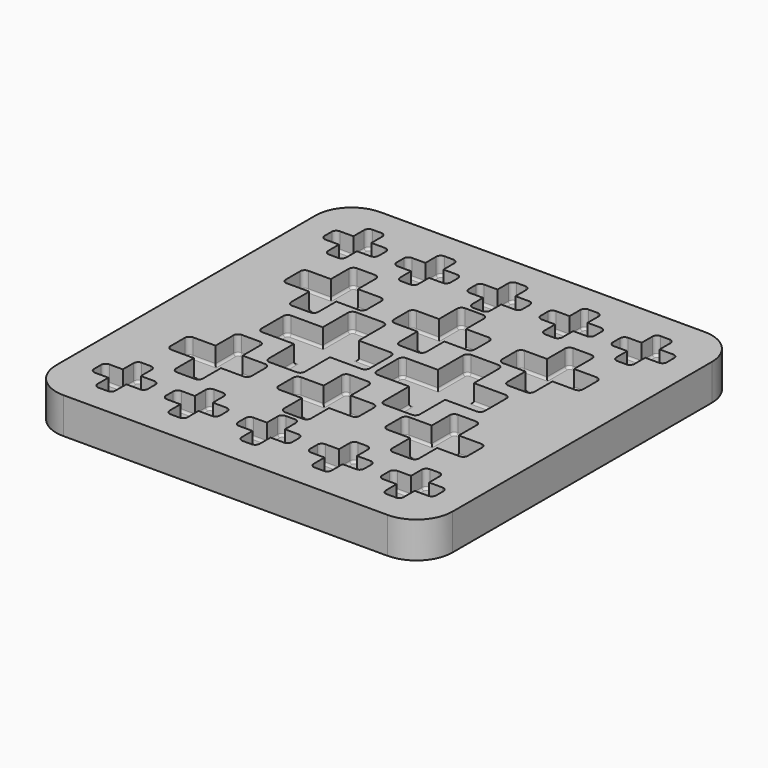
from build123d import *

# Parameters (mm, degrees)
F1_DEPTH = 6.35
F2_W     = 3.175
F2_H     = 3.175
F2_W_2   = 4.7625
F2_H_2   = 4.7625
F2_W_3   = 6.35
F2_H_3   = 6.35
F3_DEPTH = 3.175
F4_R     = 0.396875


with BuildPart() as f1:
    # F0 (on Top) → F1 (new body)
    with BuildSketch(Plane.XY):
        with BuildLine():
            Line((28.575, 34.925), (-28.575, 34.925))
            ThreePointArc((-28.575, 34.925), (-33.0651280605, 33.0651280605), (-34.925, 28.575))
            Line((-34.925, 28.575), (-34.925, -28.575))
            ThreePointArc((-34.925, -28.575), (-33.0651280605, -33.0651280605), (-28.575, -34.925))
            Line((-28.575, -34.925), (28.575, -34.925))
            ThreePointArc((28.575, -34.925), (33.0651280605, -33.0651280605), (34.925, -28.575))
            Line((34.925, -28.575), (34.925, 28.575))
            ThreePointArc((34.925, 28.575), (33.0651280605, 33.0651280605), (28.575, 34.925))
        make_face()
    extrude(amount=F1_DEPTH)

    # F2 (on face) → F3 (cut)
    with BuildSketch(Plane.XY.offset(6.35)):
        with BuildLine():
            ThreePointArc((-23.8125, 29.36875), (-24.0449839924, 29.9300160076), (-24.60625, 30.1625))
            Line((-24.60625, 30.1625), (-26.19375, 30.1625))
            ThreePointArc((-26.19375, 30.1625), (-26.7550160076, 29.9300160076), (-26.9875, 29.36875))
            Line((-26.9875, 29.36875), (-26.9875, 26.9875))
            Line((-26.9875, 26.9875), (-23.8125, 26.9875))
            Line((-23.8125, 26.9875), (-23.8125, 29.36875))
        make_face()
        with BuildLine():
            Line((-21.43125, 26.9875), (-23.8125, 26.9875))
            Line((-23.8125, 26.9875), (-23.8125, 23.8125))
            Line((-23.8125, 23.8125), (-21.43125, 23.8125))
            ThreePointArc((-21.43125, 23.8125), (-20.8699839924, 24.0449839924), (-20.6375, 24.60625))
            Line((-20.6375, 24.60625), (-20.6375, 26.19375))
            ThreePointArc((-20.6375, 26.19375), (-20.8699839924, 26.7550160076), (-21.43125, 26.9875))
        make_face()
        with Locations((-25.4, 25.4)):
            Rectangle(F2_W, F2_H)
        with BuildLine():
            Line((-26.9875, 23.8125), (-26.9875, 26.9875))
            Line((-26.9875, 26.9875), (-29.36875, 26.9875))
            ThreePointArc((-29.36875, 26.9875), (-29.9300160076, 26.7550160076), (-30.1625, 26.19375))
            Line((-30.1625, 26.19375), (-30.1625, 24.60625))
            ThreePointArc((-30.1625, 24.60625), (-29.9300160076, 24.0449839924), (-29.36875, 23.8125))
            Line((-29.36875, 23.8125), (-26.9875, 23.8125))
        make_face()
        with BuildLine():
            Line((-23.8125, 21.43125), (-23.8125, 23.8125))
            Line((-23.8125, 23.8125), (-26.9875, 23.8125))
            Line((-26.9875, 23.8125), (-26.9875, 21.43125))
            ThreePointArc((-26.9875, 21.43125), (-26.7550160076, 20.8699839924), (-26.19375, 20.6375))
            Line((-26.19375, 20.6375), (-24.60625, 20.6375))
            ThreePointArc((-24.60625, 20.6375), (-24.0449839924, 20.8699839924), (-23.8125, 21.43125))
        make_face()
        with BuildLine():
            ThreePointArc((-16.66875, 19.05), (-16.9012339924, 19.6112660076), (-17.4625, 19.84375))
            Line((-17.4625, 19.84375), (-20.6375, 19.84375))
            ThreePointArc((-20.6375, 19.84375), (-21.1987660076, 19.6112660076), (-21.43125, 19.05))
            Line((-21.43125, 19.05), (-21.43125, 15.08125))
            Line((-21.43125, 15.08125), (-16.66875, 15.08125))
            Line((-16.66875, 15.08125), (-16.66875, 19.05))
        make_face()
        with BuildLine():
            Line((-12.7, 15.08125), (-16.66875, 15.08125))
            Line((-16.66875, 15.08125), (-16.66875, 10.31875))
            Line((-16.66875, 10.31875), (-12.7, 10.31875))
            ThreePointArc((-12.7, 10.31875), (-12.1387339924, 10.5512339924), (-11.90625, 11.1125))
            Line((-11.90625, 11.1125), (-11.90625, 14.2875))
            ThreePointArc((-11.90625, 14.2875), (-12.1387339924, 14.8487660076), (-12.7, 15.08125))
        make_face()
        with Locations((-19.05, 12.7)):
            Rectangle(F2_W_2, F2_H_2)
        with BuildLine():
            Line((-21.43125, 10.31875), (-21.43125, 15.08125))
            Line((-21.43125, 15.08125), (-25.4, 15.08125))
            ThreePointArc((-25.4, 15.08125), (-25.9612660076, 14.8487660076), (-26.19375, 14.2875))
            Line((-26.19375, 14.2875), (-26.19375, 11.1125))
            ThreePointArc((-26.19375, 11.1125), (-25.9612660076, 10.5512339924), (-25.4, 10.31875))
            Line((-25.4, 10.31875), (-21.43125, 10.31875))
        make_face()
        with BuildLine():
            Line((-16.66875, 6.35), (-16.66875, 10.31875))
            Line((-16.66875, 10.31875), (-21.43125, 10.31875))
            Line((-21.43125, 10.31875), (-21.43125, 6.35))
            ThreePointArc((-21.43125, 6.35), (-21.1987660076, 5.7887339924), (-20.6375, 5.55625))
            Line((-20.6375, 5.55625), (-17.4625, 5.55625))
            ThreePointArc((-17.4625, 5.55625), (-16.9012339924, 5.7887339924), (-16.66875, 6.35))
        make_face()
        with BuildLine():
            Line((-7.77875, 9.525), (-12.54125, 9.525))
            ThreePointArc((-12.54125, 9.525), (-13.1025160076, 9.2925160076), (-13.335, 8.73125))
            Line((-13.335, 8.73125), (-13.335, 3.175))
            Line((-13.335, 3.175), (-6.985, 3.175))
            Line((-6.985, 3.175), (-6.985, 8.73125))
            ThreePointArc((-6.985, 8.73125), (-7.2174839924, 9.2925160076), (-7.77875, 9.525))
        make_face()
        with Locations((-10.16, 0)):
            Rectangle(F2_W_3, F2_H_3)
        with BuildLine():
            Line((-13.335, -3.175), (-13.335, 3.175))
            Line((-13.335, 3.175), (-18.89125, 3.175))
            ThreePointArc((-18.89125, 3.175), (-19.4525160076, 2.9425160076), (-19.685, 2.38125))
            Line((-19.685, 2.38125), (-19.685, -2.38125))
            ThreePointArc((-19.685, -2.38125), (-19.4525160076, -2.9425160076), (-18.89125, -3.175))
            Line((-18.89125, -3.175), (-13.335, -3.175))
        make_face()
        with BuildLine():
            Line((-1.42875, 3.175), (-6.985, 3.175))
            Line((-6.985, 3.175), (-6.985, -3.175))
            Line((-6.985, -3.175), (-1.42875, -3.175))
            ThreePointArc((-1.42875, -3.175), (-0.8674839924, -2.9425160076), (-0.635, -2.38125))
            Line((-0.635, -2.38125), (-0.635, 2.38125))
            ThreePointArc((-0.635, 2.38125), (-0.8674839924, 2.9425160076), (-1.42875, 3.175))
        make_face()
        with BuildLine():
            Line((-6.985, -3.175), (-13.335, -3.175))
            Line((-13.335, -3.175), (-13.335, -8.73125))
            ThreePointArc((-13.335, -8.73125), (-13.1025160076, -9.2925160076), (-12.54125, -9.525))
            Line((-12.54125, -9.525), (-7.77875, -9.525))
            ThreePointArc((-7.77875, -9.525), (-7.2174839924, -9.2925160076), (-6.985, -8.73125))
            Line((-6.985, -8.73125), (-6.985, -3.175))
        make_face()
        with BuildLine():
            ThreePointArc((-13.49375, 30.1625), (-14.0550160076, 29.9300160076), (-14.2875, 29.36875))
            Line((-14.2875, 29.36875), (-14.2875, 26.9875))
            Line((-14.2875, 26.9875), (-11.1125, 26.9875))
            Line((-11.1125, 26.9875), (-11.1125, 29.36875))
            ThreePointArc((-11.1125, 29.36875), (-11.3449839924, 29.9300160076), (-11.90625, 30.1625))
            Line((-11.90625, 30.1625), (-13.49375, 30.1625))
        make_face()
        with Locations((-12.7, 25.4)):
            Rectangle(F2_W, F2_H)
        with BuildLine():
            Line((-14.2875, 23.8125), (-14.2875, 26.9875))
            Line((-14.2875, 26.9875), (-16.66875, 26.9875))
            ThreePointArc((-16.66875, 26.9875), (-17.2300160076, 26.7550160076), (-17.4625, 26.19375))
            Line((-17.4625, 26.19375), (-17.4625, 24.60625))
            ThreePointArc((-17.4625, 24.60625), (-17.2300160076, 24.0449839924), (-16.66875, 23.8125))
            Line((-16.66875, 23.8125), (-14.2875, 23.8125))
        make_face()
        with BuildLine():
            Line((-11.1125, 23.8125), (-14.2875, 23.8125))
            Line((-14.2875, 23.8125), (-14.2875, 21.43125))
            ThreePointArc((-14.2875, 21.43125), (-14.0550160076, 20.8699839924), (-13.49375, 20.6375))
            Line((-13.49375, 20.6375), (-11.90625, 20.6375))
            ThreePointArc((-11.90625, 20.6375), (-11.3449839924, 20.8699839924), (-11.1125, 21.43125))
            Line((-11.1125, 21.43125), (-11.1125, 23.8125))
        make_face()
        with BuildLine():
            Line((-8.73125, 26.9875), (-11.1125, 26.9875))
            Line((-11.1125, 26.9875), (-11.1125, 23.8125))
            Line((-11.1125, 23.8125), (-8.73125, 23.8125))
            ThreePointArc((-8.73125, 23.8125), (-8.1699839924, 24.0449839924), (-7.9375, 24.60625))
            Line((-7.9375, 24.60625), (-7.9375, 26.19375))
            ThreePointArc((-7.9375, 26.19375), (-8.1699839924, 26.7550160076), (-8.73125, 26.9875))
        make_face()
        with BuildLine():
            ThreePointArc((-0.79375, 30.1625), (-1.3550160076, 29.9300160076), (-1.5875, 29.36875))
            Line((-1.5875, 29.36875), (-1.5875, 26.9875))
            Line((-1.5875, 26.9875), (1.5875, 26.9875))
            Line((1.5875, 26.9875), (1.5875, 29.36875))
            ThreePointArc((1.5875, 29.36875), (1.3550160076, 29.9300160076), (0.79375, 30.1625))
            Line((0.79375, 30.1625), (-0.79375, 30.1625))
        make_face()
        with Locations((0, 25.4)):
            Rectangle(F2_W, F2_H)
        with BuildLine():
            Line((-1.5875, 23.8125), (-1.5875, 26.9875))
            Line((-1.5875, 26.9875), (-3.96875, 26.9875))
            ThreePointArc((-3.96875, 26.9875), (-4.5300160076, 26.7550160076), (-4.7625, 26.19375))
            Line((-4.7625, 26.19375), (-4.7625, 24.60625))
            ThreePointArc((-4.7625, 24.60625), (-4.5300160076, 24.0449839924), (-3.96875, 23.8125))
            Line((-3.96875, 23.8125), (-1.5875, 23.8125))
        make_face()
        with BuildLine():
            Line((1.5875, 23.8125), (-1.5875, 23.8125))
            Line((-1.5875, 23.8125), (-1.5875, 21.43125))
            ThreePointArc((-1.5875, 21.43125), (-1.3550160076, 20.8699839924), (-0.79375, 20.6375))
            Line((-0.79375, 20.6375), (0.79375, 20.6375))
            ThreePointArc((0.79375, 20.6375), (1.3550160076, 20.8699839924), (1.5875, 21.43125))
            Line((1.5875, 21.43125), (1.5875, 23.8125))
        make_face()
        with BuildLine():
            Line((3.96875, 26.9875), (1.5875, 26.9875))
            Line((1.5875, 26.9875), (1.5875, 23.8125))
            Line((1.5875, 23.8125), (3.96875, 23.8125))
            ThreePointArc((3.96875, 23.8125), (4.5300160076, 24.0449839924), (4.7625, 24.60625))
            Line((4.7625, 24.60625), (4.7625, 26.19375))
            ThreePointArc((4.7625, 26.19375), (4.5300160076, 26.7550160076), (3.96875, 26.9875))
        make_face()
        with BuildLine():
            ThreePointArc((11.90625, 30.1625), (11.3449839924, 29.9300160076), (11.1125, 29.36875))
            Line((11.1125, 29.36875), (11.1125, 26.9875))
            Line((11.1125, 26.9875), (14.2875, 26.9875))
            Line((14.2875, 26.9875), (14.2875, 29.36875))
            ThreePointArc((14.2875, 29.36875), (14.0550160076, 29.9300160076), (13.49375, 30.1625))
            Line((13.49375, 30.1625), (11.90625, 30.1625))
        make_face()
        with Locations((12.7, 25.4)):
            Rectangle(F2_W, F2_H)
        with BuildLine():
            Line((11.1125, 23.8125), (11.1125, 26.9875))
            Line((11.1125, 26.9875), (8.73125, 26.9875))
            ThreePointArc((8.73125, 26.9875), (8.1699839924, 26.7550160076), (7.9375, 26.19375))
            Line((7.9375, 26.19375), (7.9375, 24.60625))
            ThreePointArc((7.9375, 24.60625), (8.1699839924, 24.0449839924), (8.73125, 23.8125))
            Line((8.73125, 23.8125), (11.1125, 23.8125))
        make_face()
        with BuildLine():
            Line((14.2875, 23.8125), (11.1125, 23.8125))
            Line((11.1125, 23.8125), (11.1125, 21.43125))
            ThreePointArc((11.1125, 21.43125), (11.3449839924, 20.8699839924), (11.90625, 20.6375))
            Line((11.90625, 20.6375), (13.49375, 20.6375))
            ThreePointArc((13.49375, 20.6375), (14.0550160076, 20.8699839924), (14.2875, 21.43125))
            Line((14.2875, 21.43125), (14.2875, 23.8125))
        make_face()
        with BuildLine():
            Line((16.66875, 26.9875), (14.2875, 26.9875))
            Line((14.2875, 26.9875), (14.2875, 23.8125))
            Line((14.2875, 23.8125), (16.66875, 23.8125))
            ThreePointArc((16.66875, 23.8125), (17.2300160076, 24.0449839924), (17.4625, 24.60625))
            Line((17.4625, 24.60625), (17.4625, 26.19375))
            ThreePointArc((17.4625, 26.19375), (17.2300160076, 26.7550160076), (16.66875, 26.9875))
        make_face()
        with BuildLine():
            ThreePointArc((24.60625, 30.1625), (24.0449839924, 29.9300160076), (23.8125, 29.36875))
            Line((23.8125, 29.36875), (23.8125, 26.9875))
            Line((23.8125, 26.9875), (26.9875, 26.9875))
            Line((26.9875, 26.9875), (26.9875, 29.36875))
            ThreePointArc((26.9875, 29.36875), (26.7550160076, 29.9300160076), (26.19375, 30.1625))
            Line((26.19375, 30.1625), (24.60625, 30.1625))
        make_face()
        with Locations((25.4, 25.4)):
            Rectangle(F2_W, F2_H)
        with BuildLine():
            Line((23.8125, 23.8125), (23.8125, 26.9875))
            Line((23.8125, 26.9875), (21.43125, 26.9875))
            ThreePointArc((21.43125, 26.9875), (20.8699839924, 26.7550160076), (20.6375, 26.19375))
            Line((20.6375, 26.19375), (20.6375, 24.60625))
            ThreePointArc((20.6375, 24.60625), (20.8699839924, 24.0449839924), (21.43125, 23.8125))
            Line((21.43125, 23.8125), (23.8125, 23.8125))
        make_face()
        with BuildLine():
            Line((26.9875, 23.8125), (23.8125, 23.8125))
            Line((23.8125, 23.8125), (23.8125, 21.43125))
            ThreePointArc((23.8125, 21.43125), (24.0449839924, 20.8699839924), (24.60625, 20.6375))
            Line((24.60625, 20.6375), (26.19375, 20.6375))
            ThreePointArc((26.19375, 20.6375), (26.7550160076, 20.8699839924), (26.9875, 21.43125))
            Line((26.9875, 21.43125), (26.9875, 23.8125))
        make_face()
        with BuildLine():
            Line((29.36875, 26.9875), (26.9875, 26.9875))
            Line((26.9875, 26.9875), (26.9875, 23.8125))
            Line((26.9875, 23.8125), (29.36875, 23.8125))
            ThreePointArc((29.36875, 23.8125), (29.9300160076, 24.0449839924), (30.1625, 24.60625))
            Line((30.1625, 24.60625), (30.1625, 26.19375))
            ThreePointArc((30.1625, 26.19375), (29.9300160076, 26.7550160076), (29.36875, 26.9875))
        make_face()
        with BuildLine():
            Line((-1.5875, 5.55625), (1.5875, 5.55625))
            ThreePointArc((1.5875, 5.55625), (2.1487660076, 5.7887339924), (2.38125, 6.35))
            Line((2.38125, 6.35), (2.38125, 10.31875))
            Line((2.38125, 10.31875), (-2.38125, 10.31875))
            Line((-2.38125, 10.31875), (-2.38125, 6.35))
            ThreePointArc((-2.38125, 6.35), (-2.1487660076, 5.7887339924), (-1.5875, 5.55625))
        make_face()
        with BuildLine():
            Line((2.38125, 15.08125), (2.38125, 10.31875))
            Line((2.38125, 10.31875), (6.35, 10.31875))
            ThreePointArc((6.35, 10.31875), (6.9112660076, 10.5512339924), (7.14375, 11.1125))
            Line((7.14375, 11.1125), (7.14375, 14.2875))
            ThreePointArc((7.14375, 14.2875), (6.9112660076, 14.8487660076), (6.35, 15.08125))
            Line((6.35, 15.08125), (2.38125, 15.08125))
        make_face()
        with Locations((0, 12.7)):
            Rectangle(F2_W_2, F2_H_2)
        with BuildLine():
            Line((-6.35, 10.31875), (-2.38125, 10.31875))
            Line((-2.38125, 10.31875), (-2.38125, 15.08125))
            Line((-2.38125, 15.08125), (-6.35, 15.08125))
            ThreePointArc((-6.35, 15.08125), (-6.9112660076, 14.8487660076), (-7.14375, 14.2875))
            Line((-7.14375, 14.2875), (-7.14375, 11.1125))
            ThreePointArc((-7.14375, 11.1125), (-6.9112660076, 10.5512339924), (-6.35, 10.31875))
        make_face()
        with BuildLine():
            Line((-2.38125, 15.08125), (2.38125, 15.08125))
            Line((2.38125, 15.08125), (2.38125, 19.05))
            ThreePointArc((2.38125, 19.05), (2.1487660076, 19.6112660076), (1.5875, 19.84375))
            Line((1.5875, 19.84375), (-1.5875, 19.84375))
            ThreePointArc((-1.5875, 19.84375), (-2.1487660076, 19.6112660076), (-2.38125, 19.05))
            Line((-2.38125, 19.05), (-2.38125, 15.08125))
        make_face()
        with BuildLine():
            Line((17.4625, 5.55625), (20.6375, 5.55625))
            ThreePointArc((20.6375, 5.55625), (21.1987660076, 5.7887339924), (21.43125, 6.35))
            Line((21.43125, 6.35), (21.43125, 10.31875))
            Line((21.43125, 10.31875), (16.66875, 10.31875))
            Line((16.66875, 10.31875), (16.66875, 6.35))
            ThreePointArc((16.66875, 6.35), (16.9012339924, 5.7887339924), (17.4625, 5.55625))
        make_face()
        with BuildLine():
            Line((21.43125, 15.08125), (21.43125, 10.31875))
            Line((21.43125, 10.31875), (25.4, 10.31875))
            ThreePointArc((25.4, 10.31875), (25.9612660076, 10.5512339924), (26.19375, 11.1125))
            Line((26.19375, 11.1125), (26.19375, 14.2875))
            ThreePointArc((26.19375, 14.2875), (25.9612660076, 14.8487660076), (25.4, 15.08125))
            Line((25.4, 15.08125), (21.43125, 15.08125))
        make_face()
        with Locations((19.05, 12.7)):
            Rectangle(F2_W_2, F2_H_2)
        with BuildLine():
            Line((12.7, 10.31875), (16.66875, 10.31875))
            Line((16.66875, 10.31875), (16.66875, 15.08125))
            Line((16.66875, 15.08125), (12.7, 15.08125))
            ThreePointArc((12.7, 15.08125), (12.1387339924, 14.8487660076), (11.90625, 14.2875))
            Line((11.90625, 14.2875), (11.90625, 11.1125))
            ThreePointArc((11.90625, 11.1125), (12.1387339924, 10.5512339924), (12.7, 10.31875))
        make_face()
        with BuildLine():
            Line((16.66875, 15.08125), (21.43125, 15.08125))
            Line((21.43125, 15.08125), (21.43125, 19.05))
            ThreePointArc((21.43125, 19.05), (21.1987660076, 19.6112660076), (20.6375, 19.84375))
            Line((20.6375, 19.84375), (17.4625, 19.84375))
            ThreePointArc((17.4625, 19.84375), (16.9012339924, 19.6112660076), (16.66875, 19.05))
            Line((16.66875, 19.05), (16.66875, 15.08125))
        make_face()
        with BuildLine():
            Line((13.3096, 3.175), (13.3096, 8.73125))
            ThreePointArc((13.3096, 8.73125), (13.0771160076, 9.2925160076), (12.51585, 9.525))
            Line((12.51585, 9.525), (7.75335, 9.525))
            ThreePointArc((7.75335, 9.525), (7.1920839924, 9.2925160076), (6.9596, 8.73125))
            Line((6.9596, 8.73125), (6.9596, 3.175))
            Line((6.9596, 3.175), (13.3096, 3.175))
        make_face()
        with BuildLine():
            Line((18.86585, 3.175), (13.3096, 3.175))
            Line((13.3096, 3.175), (13.3096, -3.175))
            Line((13.3096, -3.175), (18.86585, -3.175))
            ThreePointArc((18.86585, -3.175), (19.4271160076, -2.9425160076), (19.6596, -2.38125))
            Line((19.6596, -2.38125), (19.6596, 2.38125))
            ThreePointArc((19.6596, 2.38125), (19.4271160076, 2.9425160076), (18.86585, 3.175))
        make_face()
        with Locations((10.1346, 0)):
            Rectangle(F2_W_3, F2_H_3)
        with BuildLine():
            Line((13.3096, -8.73125), (13.3096, -3.175))
            Line((13.3096, -3.175), (6.9596, -3.175))
            Line((6.9596, -3.175), (6.9596, -8.73125))
            ThreePointArc((6.9596, -8.73125), (7.1920839924, -9.2925160076), (7.75335, -9.525))
            Line((7.75335, -9.525), (12.51585, -9.525))
            ThreePointArc((12.51585, -9.525), (13.0771160076, -9.2925160076), (13.3096, -8.73125))
        make_face()
        with BuildLine():
            Line((6.9596, -3.175), (6.9596, 3.175))
            Line((6.9596, 3.175), (1.40335, 3.175))
            ThreePointArc((1.40335, 3.175), (0.8420839924, 2.9425160076), (0.6096, 2.38125))
            Line((0.6096, 2.38125), (0.6096, -2.38125))
            ThreePointArc((0.6096, -2.38125), (0.8420839924, -2.9425160076), (1.40335, -3.175))
            Line((1.40335, -3.175), (6.9596, -3.175))
        make_face()
        with BuildLine():
            ThreePointArc((-25.4, -10.31875), (-25.9612660076, -10.5512339924), (-26.19375, -11.1125))
            Line((-26.19375, -11.1125), (-26.19375, -14.2875))
            ThreePointArc((-26.19375, -14.2875), (-25.9612660076, -14.8487660076), (-25.4, -15.08125))
            Line((-25.4, -15.08125), (-21.43125, -15.08125))
            Line((-21.43125, -15.08125), (-21.43125, -10.31875))
            Line((-21.43125, -10.31875), (-25.4, -10.31875))
        make_face()
        with BuildLine():
            Line((-21.43125, -6.35), (-21.43125, -10.31875))
            Line((-21.43125, -10.31875), (-16.66875, -10.31875))
            Line((-16.66875, -10.31875), (-16.66875, -6.35))
            ThreePointArc((-16.66875, -6.35), (-16.9012339924, -5.7887339924), (-17.4625, -5.55625))
            Line((-17.4625, -5.55625), (-20.6375, -5.55625))
            ThreePointArc((-20.6375, -5.55625), (-21.1987660076, -5.7887339924), (-21.43125, -6.35))
        make_face()
        with Locations((-19.05, -12.7)):
            Rectangle(F2_W_2, F2_H_2)
        with BuildLine():
            Line((-12.7, -10.31875), (-16.66875, -10.31875))
            Line((-16.66875, -10.31875), (-16.66875, -15.08125))
            Line((-16.66875, -15.08125), (-12.7, -15.08125))
            ThreePointArc((-12.7, -15.08125), (-12.1387339924, -14.8487660076), (-11.90625, -14.2875))
            Line((-11.90625, -14.2875), (-11.90625, -11.1125))
            ThreePointArc((-11.90625, -11.1125), (-12.1387339924, -10.5512339924), (-12.7, -10.31875))
        make_face()
        with BuildLine():
            Line((-16.66875, -15.08125), (-21.43125, -15.08125))
            Line((-21.43125, -15.08125), (-21.43125, -19.05))
            ThreePointArc((-21.43125, -19.05), (-21.1987660076, -19.6112660076), (-20.6375, -19.84375))
            Line((-20.6375, -19.84375), (-17.4625, -19.84375))
            ThreePointArc((-17.4625, -19.84375), (-16.9012339924, -19.6112660076), (-16.66875, -19.05))
            Line((-16.66875, -19.05), (-16.66875, -15.08125))
        make_face()
        with BuildLine():
            ThreePointArc((-26.9875, -29.36875), (-26.7550160076, -29.9300160076), (-26.19375, -30.1625))
            Line((-26.19375, -30.1625), (-24.60625, -30.1625))
            ThreePointArc((-24.60625, -30.1625), (-24.0449839924, -29.9300160076), (-23.8125, -29.36875))
            Line((-23.8125, -29.36875), (-23.8125, -26.9875))
            Line((-23.8125, -26.9875), (-26.9875, -26.9875))
            Line((-26.9875, -26.9875), (-26.9875, -29.36875))
        make_face()
        with Locations((-25.4, -25.4)):
            Rectangle(F2_W, F2_H)
        with BuildLine():
            Line((-29.36875, -26.9875), (-26.9875, -26.9875))
            Line((-26.9875, -26.9875), (-26.9875, -23.8125))
            Line((-26.9875, -23.8125), (-29.36875, -23.8125))
            ThreePointArc((-29.36875, -23.8125), (-29.9300160076, -24.0449839924), (-30.1625, -24.60625))
            Line((-30.1625, -24.60625), (-30.1625, -26.19375))
            ThreePointArc((-30.1625, -26.19375), (-29.9300160076, -26.7550160076), (-29.36875, -26.9875))
        make_face()
        with BuildLine():
            Line((-23.8125, -23.8125), (-23.8125, -26.9875))
            Line((-23.8125, -26.9875), (-21.43125, -26.9875))
            ThreePointArc((-21.43125, -26.9875), (-20.8699839924, -26.7550160076), (-20.6375, -26.19375))
            Line((-20.6375, -26.19375), (-20.6375, -24.60625))
            ThreePointArc((-20.6375, -24.60625), (-20.8699839924, -24.0449839924), (-21.43125, -23.8125))
            Line((-21.43125, -23.8125), (-23.8125, -23.8125))
        make_face()
        with BuildLine():
            Line((-26.9875, -21.43125), (-26.9875, -23.8125))
            Line((-26.9875, -23.8125), (-23.8125, -23.8125))
            Line((-23.8125, -23.8125), (-23.8125, -21.43125))
            ThreePointArc((-23.8125, -21.43125), (-24.0449839924, -20.8699839924), (-24.60625, -20.6375))
            Line((-24.60625, -20.6375), (-26.19375, -20.6375))
            ThreePointArc((-26.19375, -20.6375), (-26.7550160076, -20.8699839924), (-26.9875, -21.43125))
        make_face()
        with BuildLine():
            ThreePointArc((-11.90625, -30.1625), (-11.3449839924, -29.9300160076), (-11.1125, -29.36875))
            Line((-11.1125, -29.36875), (-11.1125, -26.9875))
            Line((-11.1125, -26.9875), (-14.2875, -26.9875))
            Line((-14.2875, -26.9875), (-14.2875, -29.36875))
            ThreePointArc((-14.2875, -29.36875), (-14.0550160076, -29.9300160076), (-13.49375, -30.1625))
            Line((-13.49375, -30.1625), (-11.90625, -30.1625))
        make_face()
        with Locations((-12.7, -25.4)):
            Rectangle(F2_W, F2_H)
        with BuildLine():
            Line((-11.1125, -23.8125), (-11.1125, -26.9875))
            Line((-11.1125, -26.9875), (-8.73125, -26.9875))
            ThreePointArc((-8.73125, -26.9875), (-8.1699839924, -26.7550160076), (-7.9375, -26.19375))
            Line((-7.9375, -26.19375), (-7.9375, -24.60625))
            ThreePointArc((-7.9375, -24.60625), (-8.1699839924, -24.0449839924), (-8.73125, -23.8125))
            Line((-8.73125, -23.8125), (-11.1125, -23.8125))
        make_face()
        with BuildLine():
            Line((-14.2875, -23.8125), (-11.1125, -23.8125))
            Line((-11.1125, -23.8125), (-11.1125, -21.43125))
            ThreePointArc((-11.1125, -21.43125), (-11.3449839924, -20.8699839924), (-11.90625, -20.6375))
            Line((-11.90625, -20.6375), (-13.49375, -20.6375))
            ThreePointArc((-13.49375, -20.6375), (-14.0550160076, -20.8699839924), (-14.2875, -21.43125))
            Line((-14.2875, -21.43125), (-14.2875, -23.8125))
        make_face()
        with BuildLine():
            Line((-16.66875, -26.9875), (-14.2875, -26.9875))
            Line((-14.2875, -26.9875), (-14.2875, -23.8125))
            Line((-14.2875, -23.8125), (-16.66875, -23.8125))
            ThreePointArc((-16.66875, -23.8125), (-17.2300160076, -24.0449839924), (-17.4625, -24.60625))
            Line((-17.4625, -24.60625), (-17.4625, -26.19375))
            ThreePointArc((-17.4625, -26.19375), (-17.2300160076, -26.7550160076), (-16.66875, -26.9875))
        make_face()
        with BuildLine():
            ThreePointArc((30.1625, -24.60625), (29.9300160076, -24.0449839924), (29.36875, -23.8125))
            Line((29.36875, -23.8125), (26.9875, -23.8125))
            Line((26.9875, -23.8125), (26.9875, -26.9875))
            Line((26.9875, -26.9875), (29.36875, -26.9875))
            ThreePointArc((29.36875, -26.9875), (29.9300160076, -26.7550160076), (30.1625, -26.19375))
            Line((30.1625, -26.19375), (30.1625, -24.60625))
        make_face()
        with Locations((25.4, -25.4)):
            Rectangle(F2_W, F2_H)
        with BuildLine():
            Line((23.8125, -23.8125), (26.9875, -23.8125))
            Line((26.9875, -23.8125), (26.9875, -21.43125))
            ThreePointArc((26.9875, -21.43125), (26.7550160076, -20.8699839924), (26.19375, -20.6375))
            Line((26.19375, -20.6375), (24.60625, -20.6375))
            ThreePointArc((24.60625, -20.6375), (24.0449839924, -20.8699839924), (23.8125, -21.43125))
            Line((23.8125, -21.43125), (23.8125, -23.8125))
        make_face()
        with BuildLine():
            Line((23.8125, -26.9875), (23.8125, -23.8125))
            Line((23.8125, -23.8125), (21.43125, -23.8125))
            ThreePointArc((21.43125, -23.8125), (20.8699839924, -24.0449839924), (20.6375, -24.60625))
            Line((20.6375, -24.60625), (20.6375, -26.19375))
            ThreePointArc((20.6375, -26.19375), (20.8699839924, -26.7550160076), (21.43125, -26.9875))
            Line((21.43125, -26.9875), (23.8125, -26.9875))
        make_face()
        with BuildLine():
            Line((26.9875, -29.36875), (26.9875, -26.9875))
            Line((26.9875, -26.9875), (23.8125, -26.9875))
            Line((23.8125, -26.9875), (23.8125, -29.36875))
            ThreePointArc((23.8125, -29.36875), (24.0449839924, -29.9300160076), (24.60625, -30.1625))
            Line((24.60625, -30.1625), (26.19375, -30.1625))
            ThreePointArc((26.19375, -30.1625), (26.7550160076, -29.9300160076), (26.9875, -29.36875))
        make_face()
        with BuildLine():
            ThreePointArc((-2.38125, -19.05), (-2.1487660076, -19.6112660076), (-1.5875, -19.84375))
            Line((-1.5875, -19.84375), (1.5875, -19.84375))
            ThreePointArc((1.5875, -19.84375), (2.1487660076, -19.6112660076), (2.38125, -19.05))
            Line((2.38125, -19.05), (2.38125, -15.08125))
            Line((2.38125, -15.08125), (-2.38125, -15.08125))
            Line((-2.38125, -15.08125), (-2.38125, -19.05))
        make_face()
        with Locations((0, -12.7)):
            Rectangle(F2_W_2, F2_H_2)
        with BuildLine():
            Line((-6.35, -15.08125), (-2.38125, -15.08125))
            Line((-2.38125, -15.08125), (-2.38125, -10.31875))
            Line((-2.38125, -10.31875), (-6.35, -10.31875))
            ThreePointArc((-6.35, -10.31875), (-6.9112660076, -10.5512339924), (-7.14375, -11.1125))
            Line((-7.14375, -11.1125), (-7.14375, -14.2875))
            ThreePointArc((-7.14375, -14.2875), (-6.9112660076, -14.8487660076), (-6.35, -15.08125))
        make_face()
        with BuildLine():
            Line((2.38125, -10.31875), (2.38125, -15.08125))
            Line((2.38125, -15.08125), (6.35, -15.08125))
            ThreePointArc((6.35, -15.08125), (6.9112660076, -14.8487660076), (7.14375, -14.2875))
            Line((7.14375, -14.2875), (7.14375, -11.1125))
            ThreePointArc((7.14375, -11.1125), (6.9112660076, -10.5512339924), (6.35, -10.31875))
            Line((6.35, -10.31875), (2.38125, -10.31875))
        make_face()
        with BuildLine():
            Line((-2.38125, -6.35), (-2.38125, -10.31875))
            Line((-2.38125, -10.31875), (2.38125, -10.31875))
            Line((2.38125, -10.31875), (2.38125, -6.35))
            ThreePointArc((2.38125, -6.35), (2.1487660076, -5.7887339924), (1.5875, -5.55625))
            Line((1.5875, -5.55625), (-1.5875, -5.55625))
            ThreePointArc((-1.5875, -5.55625), (-2.1487660076, -5.7887339924), (-2.38125, -6.35))
        make_face()
        with BuildLine():
            ThreePointArc((11.1125, -29.36875), (11.3449839924, -29.9300160076), (11.90625, -30.1625))
            Line((11.90625, -30.1625), (13.49375, -30.1625))
            ThreePointArc((13.49375, -30.1625), (14.0550160076, -29.9300160076), (14.2875, -29.36875))
            Line((14.2875, -29.36875), (14.2875, -26.9875))
            Line((14.2875, -26.9875), (11.1125, -26.9875))
            Line((11.1125, -26.9875), (11.1125, -29.36875))
        make_face()
        with Locations((12.7, -25.4)):
            Rectangle(F2_W, F2_H)
        with BuildLine():
            Line((8.73125, -26.9875), (11.1125, -26.9875))
            Line((11.1125, -26.9875), (11.1125, -23.8125))
            Line((11.1125, -23.8125), (8.73125, -23.8125))
            ThreePointArc((8.73125, -23.8125), (8.1699839924, -24.0449839924), (7.9375, -24.60625))
            Line((7.9375, -24.60625), (7.9375, -26.19375))
            ThreePointArc((7.9375, -26.19375), (8.1699839924, -26.7550160076), (8.73125, -26.9875))
        make_face()
        with BuildLine():
            Line((14.2875, -23.8125), (14.2875, -26.9875))
            Line((14.2875, -26.9875), (16.66875, -26.9875))
            ThreePointArc((16.66875, -26.9875), (17.2300160076, -26.7550160076), (17.4625, -26.19375))
            Line((17.4625, -26.19375), (17.4625, -24.60625))
            ThreePointArc((17.4625, -24.60625), (17.2300160076, -24.0449839924), (16.66875, -23.8125))
            Line((16.66875, -23.8125), (14.2875, -23.8125))
        make_face()
        with BuildLine():
            Line((11.1125, -21.43125), (11.1125, -23.8125))
            Line((11.1125, -23.8125), (14.2875, -23.8125))
            Line((14.2875, -23.8125), (14.2875, -21.43125))
            ThreePointArc((14.2875, -21.43125), (14.0550160076, -20.8699839924), (13.49375, -20.6375))
            Line((13.49375, -20.6375), (11.90625, -20.6375))
            ThreePointArc((11.90625, -20.6375), (11.3449839924, -20.8699839924), (11.1125, -21.43125))
        make_face()
        with BuildLine():
            ThreePointArc((-1.5875, -29.36875), (-1.3550160076, -29.9300160076), (-0.79375, -30.1625))
            Line((-0.79375, -30.1625), (0.79375, -30.1625))
            ThreePointArc((0.79375, -30.1625), (1.3550160076, -29.9300160076), (1.5875, -29.36875))
            Line((1.5875, -29.36875), (1.5875, -26.9875))
            Line((1.5875, -26.9875), (-1.5875, -26.9875))
            Line((-1.5875, -26.9875), (-1.5875, -29.36875))
        make_face()
        with BuildLine():
            Line((-3.96875, -26.9875), (-1.5875, -26.9875))
            Line((-1.5875, -26.9875), (-1.5875, -23.8125))
            Line((-1.5875, -23.8125), (-3.96875, -23.8125))
            ThreePointArc((-3.96875, -23.8125), (-4.5300160076, -24.0449839924), (-4.7625, -24.60625))
            Line((-4.7625, -24.60625), (-4.7625, -26.19375))
            ThreePointArc((-4.7625, -26.19375), (-4.5300160076, -26.7550160076), (-3.96875, -26.9875))
        make_face()
        with Locations((0, -25.4)):
            Rectangle(F2_W, F2_H)
        with BuildLine():
            Line((-1.5875, -21.43125), (-1.5875, -23.8125))
            Line((-1.5875, -23.8125), (1.5875, -23.8125))
            Line((1.5875, -23.8125), (1.5875, -21.43125))
            ThreePointArc((1.5875, -21.43125), (1.3550160076, -20.8699839924), (0.79375, -20.6375))
            Line((0.79375, -20.6375), (-0.79375, -20.6375))
            ThreePointArc((-0.79375, -20.6375), (-1.3550160076, -20.8699839924), (-1.5875, -21.43125))
        make_face()
        with BuildLine():
            Line((1.5875, -23.8125), (1.5875, -26.9875))
            Line((1.5875, -26.9875), (3.96875, -26.9875))
            ThreePointArc((3.96875, -26.9875), (4.5300160076, -26.7550160076), (4.7625, -26.19375))
            Line((4.7625, -26.19375), (4.7625, -24.60625))
            ThreePointArc((4.7625, -24.60625), (4.5300160076, -24.0449839924), (3.96875, -23.8125))
            Line((3.96875, -23.8125), (1.5875, -23.8125))
        make_face()
        with BuildLine():
            ThreePointArc((26.19375, -11.1125), (25.9612660076, -10.5512339924), (25.4, -10.31875))
            Line((25.4, -10.31875), (21.43125, -10.31875))
            Line((21.43125, -10.31875), (21.43125, -15.08125))
            Line((21.43125, -15.08125), (25.4, -15.08125))
            ThreePointArc((25.4, -15.08125), (25.9612660076, -14.8487660076), (26.19375, -14.2875))
            Line((26.19375, -14.2875), (26.19375, -11.1125))
        make_face()
        with BuildLine():
            Line((16.66875, -10.31875), (21.43125, -10.31875))
            Line((21.43125, -10.31875), (21.43125, -6.35))
            ThreePointArc((21.43125, -6.35), (21.1987660076, -5.7887339924), (20.6375, -5.55625))
            Line((20.6375, -5.55625), (17.4625, -5.55625))
            ThreePointArc((17.4625, -5.55625), (16.9012339924, -5.7887339924), (16.66875, -6.35))
            Line((16.66875, -6.35), (16.66875, -10.31875))
        make_face()
        with Locations((19.05, -12.7)):
            Rectangle(F2_W_2, F2_H_2)
        with BuildLine():
            Line((21.43125, -19.05), (21.43125, -15.08125))
            Line((21.43125, -15.08125), (16.66875, -15.08125))
            Line((16.66875, -15.08125), (16.66875, -19.05))
            ThreePointArc((16.66875, -19.05), (16.9012339924, -19.6112660076), (17.4625, -19.84375))
            Line((17.4625, -19.84375), (20.6375, -19.84375))
            ThreePointArc((20.6375, -19.84375), (21.1987660076, -19.6112660076), (21.43125, -19.05))
        make_face()
        with BuildLine():
            Line((16.66875, -15.08125), (16.66875, -10.31875))
            Line((16.66875, -10.31875), (12.7, -10.31875))
            ThreePointArc((12.7, -10.31875), (12.1387339924, -10.5512339924), (11.90625, -11.1125))
            Line((11.90625, -11.1125), (11.90625, -14.2875))
            ThreePointArc((11.90625, -14.2875), (12.1387339924, -14.8487660076), (12.7, -15.08125))
            Line((12.7, -15.08125), (16.66875, -15.08125))
        make_face()
    extrude(amount=-F3_DEPTH, mode=Mode.SUBTRACT)

    # F4
    f4_edges = [f1.edges().sort_by_distance(p)[0] for p in [
        (-24.044984, 29.930016, 3.175),
        (-25.4, 30.1625, 3.175),
        (-26.755016, 29.930016, 3.175),
        (-26.9875, 28.178125, 3.175),
        (-28.178125, 26.9875, 3.175),
        (-29.930016, 26.755016, 3.175),
        (-30.1625, 25.4, 3.175),
        (-29.930016, 24.044984, 3.175),
        (-28.178125, 23.8125, 3.175),
        (-26.9875, 22.621875, 3.175),
        (-26.755016, 20.869984, 3.175),
        (-25.4, 20.6375, 3.175),
        (-24.044984, 20.869984, 3.175),
        (-23.8125, 22.621875, 3.175),
        (-22.621875, 23.8125, 3.175),
        (-20.869984, 24.044984, 3.175),
        (-20.6375, 25.4, 3.175),
        (-20.869984, 26.755016, 3.175),
        (-22.621875, 26.9875, 3.175),
        (-23.8125, 28.178125, 3.175),
        (-14.055016, 29.930016, 3.175),
        (-14.2875, 28.178125, 3.175),
        (-15.478125, 26.9875, 3.175),
        (-17.230016, 26.755016, 3.175),
        (-17.4625, 25.4, 3.175),
        (-17.230016, 24.044984, 3.175),
        (-15.478125, 23.8125, 3.175),
        (-14.2875, 22.621875, 3.175),
        (-14.055016, 20.869984, 3.175),
        (-12.7, 20.6375, 3.175),
        (-11.344984, 20.869984, 3.175),
        (-11.1125, 22.621875, 3.175),
        (-9.921875, 23.8125, 3.175),
        (-8.169984, 24.044984, 3.175),
        (-7.9375, 25.4, 3.175),
        (-8.169984, 26.755016, 3.175),
        (-9.921875, 26.9875, 3.175),
        (-11.1125, 28.178125, 3.175),
        (-11.344984, 29.930016, 3.175),
        (-12.7, 30.1625, 3.175),
        (1.355016, 29.930016, 3.175),
        (0, 30.1625, 3.175),
        (-1.355016, 29.930016, 3.175),
        (-1.5875, 28.178125, 3.175),
        (-2.778125, 26.9875, 3.175),
        (-4.530016, 26.755016, 3.175),
        (-4.7625, 25.4, 3.175),
        (-4.530016, 24.044984, 3.175),
        (-2.778125, 23.8125, 3.175),
        (-1.5875, 22.621875, 3.175),
        (-1.355016, 20.869984, 3.175),
        (0, 20.6375, 3.175),
        (1.355016, 20.869984, 3.175),
        (1.5875, 22.621875, 3.175),
        (2.778125, 23.8125, 3.175),
        (4.530016, 24.044984, 3.175),
        (4.7625, 25.4, 3.175),
        (4.530016, 26.755016, 3.175),
        (2.778125, 26.9875, 3.175),
        (1.5875, 28.178125, 3.175),
        (11.344984, 29.930016, 3.175),
        (11.1125, 28.178125, 3.175),
        (9.921875, 26.9875, 3.175),
        (8.169984, 26.755016, 3.175),
        (7.9375, 25.4, 3.175),
        (8.169984, 24.044984, 3.175),
        (9.921875, 23.8125, 3.175),
        (11.1125, 22.621875, 3.175),
        (11.344984, 20.869984, 3.175),
        (12.7, 20.6375, 3.175),
        (14.055016, 20.869984, 3.175),
        (14.2875, 22.621875, 3.175),
        (15.478125, 23.8125, 3.175),
        (17.230016, 24.044984, 3.175),
        (17.4625, 25.4, 3.175),
        (17.230016, 26.755016, 3.175),
        (15.478125, 26.9875, 3.175),
        (14.2875, 28.178125, 3.175),
        (14.055016, 29.930016, 3.175),
        (12.7, 30.1625, 3.175),
        (24.044984, 29.930016, 3.175),
        (23.8125, 28.178125, 3.175),
        (22.621875, 26.9875, 3.175),
        (20.869984, 26.755016, 3.175),
        (20.6375, 25.4, 3.175),
        (20.869984, 24.044984, 3.175),
        (22.621875, 23.8125, 3.175),
        (23.8125, 22.621875, 3.175),
        (24.044984, 20.869984, 3.175),
        (25.4, 20.6375, 3.175),
        (26.755016, 20.869984, 3.175),
        (26.9875, 22.621875, 3.175),
        (28.178125, 23.8125, 3.175),
        (29.930016, 24.044984, 3.175),
        (30.1625, 25.4, 3.175),
        (29.930016, 26.755016, 3.175),
        (28.178125, 26.9875, 3.175),
        (26.9875, 28.178125, 3.175),
        (26.755016, 29.930016, 3.175),
        (25.4, 30.1625, 3.175),
        (19.05, 5.55625, 3.175),
        (21.198766, 5.788734, 3.175),
        (21.43125, 8.334375, 3.175),
        (23.415625, 10.31875, 3.175),
        (25.961266, 10.551234, 3.175),
        (26.19375, 12.7, 3.175),
        (25.961266, 14.848766, 3.175),
        (23.415625, 15.08125, 3.175),
        (21.43125, 17.065625, 3.175),
        (21.198766, 19.611266, 3.175),
        (19.05, 19.84375, 3.175),
        (16.901234, 19.611266, 3.175),
        (16.66875, 17.065625, 3.175),
        (14.684375, 15.08125, 3.175),
        (12.138734, 14.848766, 3.175),
        (11.90625, 12.7, 3.175),
        (12.138734, 10.551234, 3.175),
        (14.684375, 10.31875, 3.175),
        (16.66875, 8.334375, 3.175),
        (16.901234, 5.788734, 3.175),
        (-2.148766, 5.788734, 3.175),
        (0, 5.55625, 3.175),
        (2.148766, 5.788734, 3.175),
        (2.38125, 8.334375, 3.175),
        (4.365625, 10.31875, 3.175),
        (6.911266, 10.551234, 3.175),
        (7.14375, 12.7, 3.175),
        (6.911266, 14.848766, 3.175),
        (4.365625, 15.08125, 3.175),
        (2.38125, 17.065625, 3.175),
        (2.148766, 19.611266, 3.175),
        (0, 19.84375, 3.175),
        (-2.148766, 19.611266, 3.175),
        (-2.38125, 17.065625, 3.175),
        (-4.365625, 15.08125, 3.175),
        (-6.911266, 14.848766, 3.175),
        (-7.14375, 12.7, 3.175),
        (-6.911266, 10.551234, 3.175),
        (-4.365625, 10.31875, 3.175),
        (-2.38125, 8.334375, 3.175),
        (-16.901234, 19.611266, 3.175),
        (-19.05, 19.84375, 3.175),
        (-21.198766, 19.611266, 3.175),
        (-21.43125, 17.065625, 3.175),
        (-23.415625, 15.08125, 3.175),
        (-25.961266, 14.848766, 3.175),
        (-26.19375, 12.7, 3.175),
        (-25.961266, 10.551234, 3.175),
        (-23.415625, 10.31875, 3.175),
        (-21.43125, 8.334375, 3.175),
        (-21.198766, 5.788734, 3.175),
        (-19.05, 5.55625, 3.175),
        (-16.901234, 5.788734, 3.175),
        (-16.66875, 8.334375, 3.175),
        (-14.684375, 10.31875, 3.175),
        (-12.138734, 10.551234, 3.175),
        (-11.90625, 12.7, 3.175),
        (-12.138734, 14.848766, 3.175),
        (-14.684375, 15.08125, 3.175),
        (-16.66875, 17.065625, 3.175),
        (-6.985, 5.953125, 3.175),
        (-7.217484, 9.292516, 3.175),
        (-10.16, 9.525, 3.175),
        (-13.102516, 9.292516, 3.175),
        (-13.335, 5.953125, 3.175),
        (-16.113125, 3.175, 3.175),
        (-19.452516, 2.942516, 3.175),
        (-19.685, 0, 3.175),
        (-19.452516, -2.942516, 3.175),
        (-16.113125, -3.175, 3.175),
        (-13.335, -5.953125, 3.175),
        (-13.102516, -9.292516, 3.175),
        (-10.16, -9.525, 3.175),
        (-7.217484, -9.292516, 3.175),
        (-6.985, -5.953125, 3.175),
        (-4.206875, -3.175, 3.175),
        (-0.867484, -2.942516, 3.175),
        (-0.635, 0, 3.175),
        (-0.867484, 2.942516, 3.175),
        (-4.206875, 3.175, 3.175),
        (13.3096, 5.953125, 3.175),
        (13.077116, 9.292516, 3.175),
        (10.1346, 9.525, 3.175),
        (7.192084, 9.292516, 3.175),
        (6.9596, 5.953125, 3.175),
        (4.181475, 3.175, 3.175),
        (0.842084, 2.942516, 3.175),
        (0.6096, 0, 3.175),
        (0.842084, -2.942516, 3.175),
        (4.181475, -3.175, 3.175),
        (6.9596, -5.953125, 3.175),
        (7.192084, -9.292516, 3.175),
        (10.1346, -9.525, 3.175),
        (13.077116, -9.292516, 3.175),
        (13.3096, -5.953125, 3.175),
        (16.087725, -3.175, 3.175),
        (19.427116, -2.942516, 3.175),
        (19.6596, 0, 3.175),
        (19.427116, 2.942516, 3.175),
        (16.087725, 3.175, 3.175),
        (-25.961266, -10.551234, 3.175),
        (-26.19375, -12.7, 3.175),
        (-25.961266, -14.848766, 3.175),
        (-23.415625, -15.08125, 3.175),
        (-21.43125, -17.065625, 3.175),
        (-21.198766, -19.611266, 3.175),
        (-19.05, -19.84375, 3.175),
        (-16.901234, -19.611266, 3.175),
        (-16.66875, -17.065625, 3.175),
        (-14.684375, -15.08125, 3.175),
        (-12.138734, -14.848766, 3.175),
        (-11.90625, -12.7, 3.175),
        (-12.138734, -10.551234, 3.175),
        (-14.684375, -10.31875, 3.175),
        (-16.66875, -8.334375, 3.175),
        (-16.901234, -5.788734, 3.175),
        (-19.05, -5.55625, 3.175),
        (-21.198766, -5.788734, 3.175),
        (-21.43125, -8.334375, 3.175),
        (-23.415625, -10.31875, 3.175),
        (-2.38125, -17.065625, 3.175),
        (-2.148766, -19.611266, 3.175),
        (0, -19.84375, 3.175),
        (2.148766, -19.611266, 3.175),
        (2.38125, -17.065625, 3.175),
        (4.365625, -15.08125, 3.175),
        (6.911266, -14.848766, 3.175),
        (7.14375, -12.7, 3.175),
        (6.911266, -10.551234, 3.175),
        (4.365625, -10.31875, 3.175),
        (2.38125, -8.334375, 3.175),
        (2.148766, -5.788734, 3.175),
        (0, -5.55625, 3.175),
        (-2.148766, -5.788734, 3.175),
        (-2.38125, -8.334375, 3.175),
        (-4.365625, -10.31875, 3.175),
        (-6.911266, -10.551234, 3.175),
        (-7.14375, -12.7, 3.175),
        (-6.911266, -14.848766, 3.175),
        (-4.365625, -15.08125, 3.175),
        (25.961266, -14.848766, 3.175),
        (26.19375, -12.7, 3.175),
        (25.961266, -10.551234, 3.175),
        (23.415625, -10.31875, 3.175),
        (21.43125, -8.334375, 3.175),
        (21.198766, -5.788734, 3.175),
        (19.05, -5.55625, 3.175),
        (16.901234, -5.788734, 3.175),
        (16.66875, -8.334375, 3.175),
        (14.684375, -10.31875, 3.175),
        (12.138734, -10.551234, 3.175),
        (11.90625, -12.7, 3.175),
        (12.138734, -14.848766, 3.175),
        (14.684375, -15.08125, 3.175),
        (16.66875, -17.065625, 3.175),
        (16.901234, -19.611266, 3.175),
        (19.05, -19.84375, 3.175),
        (21.198766, -19.611266, 3.175),
        (21.43125, -17.065625, 3.175),
        (23.415625, -15.08125, 3.175),
        (-26.755016, -29.930016, 3.175),
        (-25.4, -30.1625, 3.175),
        (-24.044984, -29.930016, 3.175),
        (-23.8125, -28.178125, 3.175),
        (-22.621875, -26.9875, 3.175),
        (-20.869984, -26.755016, 3.175),
        (-20.6375, -25.4, 3.175),
        (-20.869984, -24.044984, 3.175),
        (-22.621875, -23.8125, 3.175),
        (-23.8125, -22.621875, 3.175),
        (-24.044984, -20.869984, 3.175),
        (-25.4, -20.6375, 3.175),
        (-26.755016, -20.869984, 3.175),
        (-26.9875, -22.621875, 3.175),
        (-28.178125, -23.8125, 3.175),
        (-29.930016, -24.044984, 3.175),
        (-30.1625, -25.4, 3.175),
        (-29.930016, -26.755016, 3.175),
        (-28.178125, -26.9875, 3.175),
        (-26.9875, -28.178125, 3.175),
        (-11.344984, -29.930016, 3.175),
        (-11.1125, -28.178125, 3.175),
        (-9.921875, -26.9875, 3.175),
        (-8.169984, -26.755016, 3.175),
        (-7.9375, -25.4, 3.175),
        (-8.169984, -24.044984, 3.175),
        (-9.921875, -23.8125, 3.175),
        (-11.1125, -22.621875, 3.175),
        (-11.344984, -20.869984, 3.175),
        (-12.7, -20.6375, 3.175),
        (-14.055016, -20.869984, 3.175),
        (-14.2875, -22.621875, 3.175),
        (-15.478125, -23.8125, 3.175),
        (-17.230016, -24.044984, 3.175),
        (-17.4625, -25.4, 3.175),
        (-17.230016, -26.755016, 3.175),
        (-15.478125, -26.9875, 3.175),
        (-14.2875, -28.178125, 3.175),
        (-14.055016, -29.930016, 3.175),
        (-12.7, -30.1625, 3.175),
        (-1.355016, -29.930016, 3.175),
        (0, -30.1625, 3.175),
        (1.355016, -29.930016, 3.175),
        (1.5875, -28.178125, 3.175),
        (2.778125, -26.9875, 3.175),
        (4.530016, -26.755016, 3.175),
        (4.7625, -25.4, 3.175),
        (4.530016, -24.044984, 3.175),
        (2.778125, -23.8125, 3.175),
        (1.5875, -22.621875, 3.175),
        (1.355016, -20.869984, 3.175),
        (0, -20.6375, 3.175),
        (-1.355016, -20.869984, 3.175),
        (-1.5875, -22.621875, 3.175),
        (-2.778125, -23.8125, 3.175),
        (-4.530016, -24.044984, 3.175),
        (-4.7625, -25.4, 3.175),
        (-4.530016, -26.755016, 3.175),
        (-2.778125, -26.9875, 3.175),
        (-1.5875, -28.178125, 3.175),
        (11.344984, -29.930016, 3.175),
        (12.7, -30.1625, 3.175),
        (14.055016, -29.930016, 3.175),
        (14.2875, -28.178125, 3.175),
        (15.478125, -26.9875, 3.175),
        (17.230016, -26.755016, 3.175),
        (17.4625, -25.4, 3.175),
        (17.230016, -24.044984, 3.175),
        (15.478125, -23.8125, 3.175),
        (14.2875, -22.621875, 3.175),
        (14.055016, -20.869984, 3.175),
        (12.7, -20.6375, 3.175),
        (11.344984, -20.869984, 3.175),
        (11.1125, -22.621875, 3.175),
        (9.921875, -23.8125, 3.175),
        (8.169984, -24.044984, 3.175),
        (7.9375, -25.4, 3.175),
        (8.169984, -26.755016, 3.175),
        (9.921875, -26.9875, 3.175),
        (11.1125, -28.178125, 3.175),
        (29.930016, -24.044984, 3.175),
        (28.178125, -23.8125, 3.175),
        (26.9875, -22.621875, 3.175),
        (26.755016, -20.869984, 3.175),
        (25.4, -20.6375, 3.175),
        (24.044984, -20.869984, 3.175),
        (23.8125, -22.621875, 3.175),
        (22.621875, -23.8125, 3.175),
        (20.869984, -24.044984, 3.175),
        (20.6375, -25.4, 3.175),
        (20.869984, -26.755016, 3.175),
        (22.621875, -26.9875, 3.175),
        (23.8125, -28.178125, 3.175),
        (24.044984, -29.930016, 3.175),
        (25.4, -30.1625, 3.175),
        (26.755016, -29.930016, 3.175),
        (26.9875, -28.178125, 3.175),
        (28.178125, -26.9875, 3.175),
        (29.930016, -26.755016, 3.175),
        (30.1625, -25.4, 3.175),
    ]]
    fillet(f4_edges, radius=F4_R)


solid = f1.part
